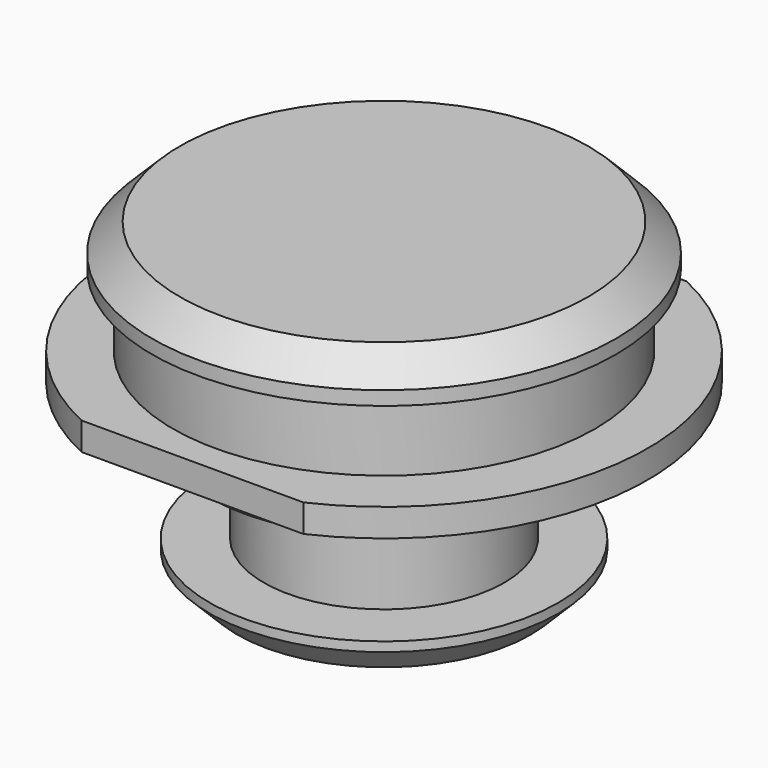
from build123d import *

# Parameters (mm, degrees)
F0_R      = 4.75
F1_DEPTH  = 0.5
F2_R      = 3.8
F3_DEPTH  = 1.3
F4_R      = 4.175
F4_R_2    = 3.8
F5_DEPTH  = 0.75
F6_SIZE   = 0.5
F8_DEPTH  = 2.551
F9_R      = 3.15
F10_DEPTH = 0.8
F11_R     = 2.165
F12_DEPTH = 1.67
F13_R     = 3.14
F14_DEPTH = 0.67
F15_SIZE  = 0.5


with BuildPart() as f1:
    # F0 (on Top) → F1 (new body)
    with BuildSketch(Plane.XY):
        Circle(F0_R)
    extrude(amount=F1_DEPTH)

    # F2 (on face) → F3 (join)
    with BuildSketch(Plane.XY.offset(0.5)):
        Circle(F2_R)
    extrude(amount=F3_DEPTH)

    # F4 (on face) → F5 (join)
    with BuildSketch(Plane.XY.offset(1.8)):
        Circle(F4_R)
        Circle(F4_R_2, mode=Mode.SUBTRACT)
        Circle(F4_R_2)
    extrude(amount=F5_DEPTH)

    # F6
    f6_edges = [f1.edges().sort_by_distance(p)[0] for p in [
        (-4.175, 0, 2.55),
    ]]
    chamfer(f6_edges, length=F6_SIZE)

    # F7 (on face) → F8 (cut, through all)
    with BuildSketch(Plane(origin=(0, 0, 0), x_dir=(1, 0, 0), z_dir=(0, 0, -1))):
        with BuildLine():
            Line((-1.9965971051, 4.31), (0, 4.31))
            Line((0, 4.31), (1.9965971051, 4.31))
            ThreePointArc((1.9965971051, 4.31), (0, 4.75), (-1.9965971051, 4.31))
        make_face()
        with BuildLine():
            Line((0, -4.31), (-1.9965971051, -4.31))
            ThreePointArc((-1.9965971051, -4.31), (0, -4.75), (1.9965971051, -4.31))
            Line((1.9965971051, -4.31), (0, -4.31))
        make_face()
    extrude(amount=-F8_DEPTH, mode=Mode.SUBTRACT)

    # F9 (on face) → F10 (join)
    with BuildSketch(Plane(origin=(0, 0, 0), x_dir=(1, 0, 0), z_dir=(0, 0, -1))):
        Circle(F9_R)
    extrude(amount=F10_DEPTH)

    # F11 (on face) → F12 (join)
    with BuildSketch(Plane(origin=(0, 0, -0.8), x_dir=(1, 0, 0), z_dir=(0, 0, -1))):
        Circle(F11_R)
    extrude(amount=F12_DEPTH)

    # F13 (on face) → F14 (join)
    with BuildSketch(Plane(origin=(0, 0, -2.47), x_dir=(1, 0, 0), z_dir=(0, 0, -1))):
        Circle(F13_R)
    extrude(amount=F14_DEPTH)

    # F15
    f15_edges = [f1.edges().sort_by_distance(p)[0] for p in [
        (-3.14, 0, -3.14),
    ]]
    chamfer(f15_edges, length=F15_SIZE)


solid = f1.part
